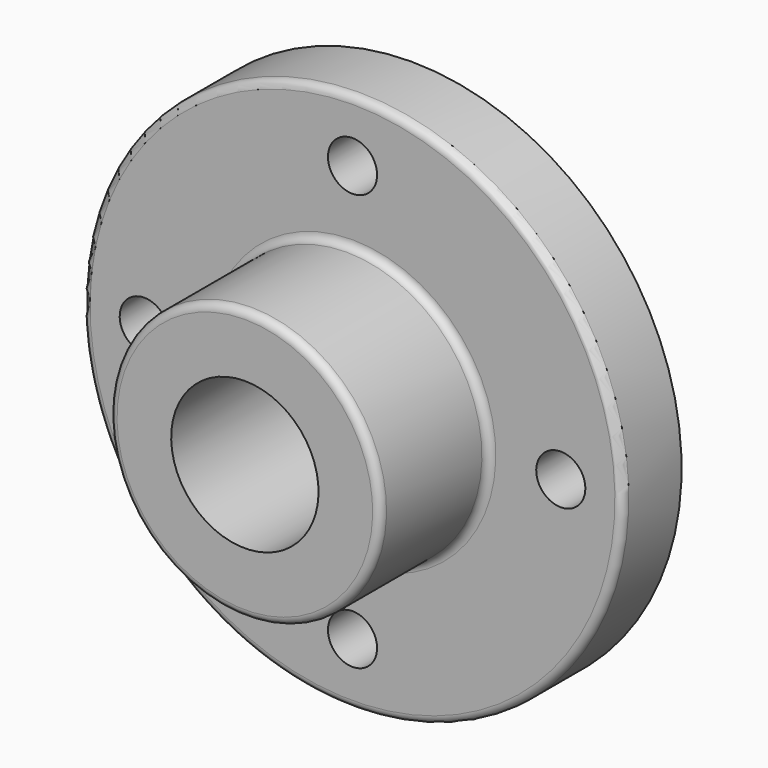
from build123d import *

# Parameters (mm, degrees)
F2_R            = 63.5
F2_R_2          = 6.35
F3_DEPTH        = 53.849
F3_COPIES_COUNT = 4
F4_R            = 2


# Not quite as in the source:
# - a pattern or mirror of a feature is missing from the dataset's text; its kind, count and spacing are read off the source's solid
# - a feature names something its author has since deleted; it is built from what else it names


with BuildPart() as f1:
    # F0 (on Right) → F1 (revolve)
    with BuildSketch(Plane.YZ):
        Polygon((-53.848, 19.05), (0, 19.05), (0, 69.85), (-19.05, 69.85), (-19.05, 35.052), (-53.848, 35.052), align=None)
    revolve(axis=Axis((0, -26.924, 0), (0, -1, 0)))

    # F2 (on Front) → F3 (cut, through all)
    with BuildSketch(Plane.XZ):
        with Locations((0, 265.2071825894)):
            Circle(F2_R)
        with Locations((0, 53.848)):
            Circle(F2_R_2)
    f3 = extrude(amount=F3_DEPTH, mode=Mode.SUBTRACT)

    # F3_copies: F3 ×4 about axis
    f3_copies_axis = Axis((0, 0, 0), (0, 1, 0))
    for i in range(1, F3_COPIES_COUNT):
        add(f3.rotate(f3_copies_axis, i * 360 / F3_COPIES_COUNT), mode=Mode.SUBTRACT)

    # F4
    f4_edges = [f1.edges().sort_by_distance(p)[0] for p in [
        (0, -19.05, -69.85),
        (0, -19.05, -35.052),
        (0, -53.848, -35.052),
    ]]
    fillet(f4_edges, radius=F4_R)


solid = f1.part
